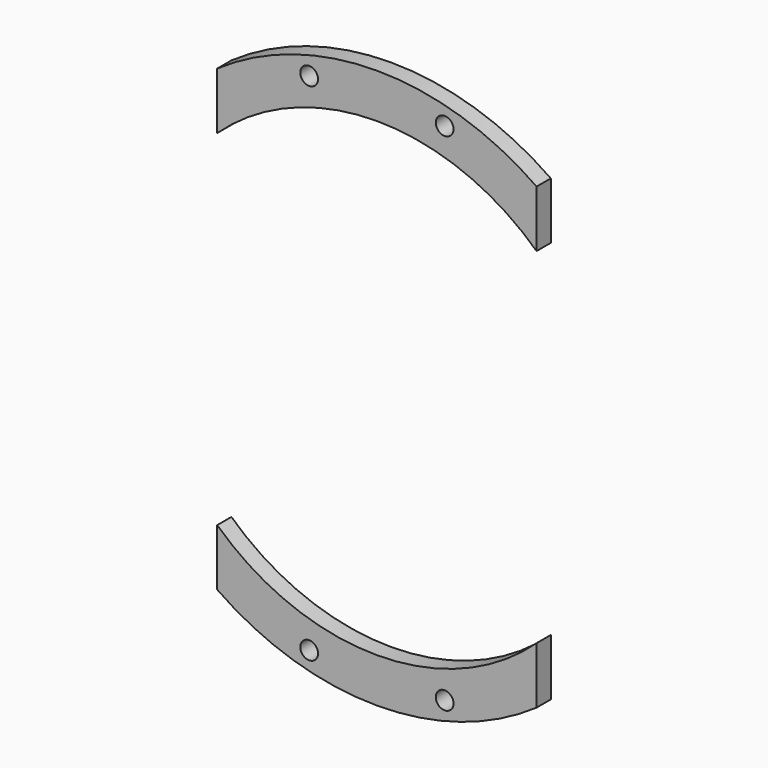
from build123d import *

# Parameters (mm, degrees)
F0_R     = 10
F1_DEPTH = 20


with BuildPart() as f1:
    # F0 (on Front) → F1 (new body)
    with BuildSketch(Plane.XZ):
        with BuildLine():
            ThreePointArc((-180, 194.4865033878), (0, 265), (180, 194.4865033878))
            Line((180, 194.4865033878), (180, 258.5053190942))
            ThreePointArc((180, 258.5053190942), (0, 315), (-180, 258.5053190942))
            Line((-180, 258.5053190942), (-180, 194.4865033878))
        make_face()
        with Locations((-76.3516183052, 284.9481187553)):
            Circle(F0_R, mode=Mode.SUBTRACT)
        with Locations((76.3516183052, 284.9481187553)):
            Circle(F0_R, mode=Mode.SUBTRACT)
    extrude(amount=F1_DEPTH)


with BuildPart() as f1b:
    # F0 (on Front) → F1, piece 2 (new body)
    with BuildSketch(Plane.XZ):
        with BuildLine():
            Line((180, -258.5053190942), (180, -194.4865033878))
            ThreePointArc((180, -194.4865033878), (0, -265), (-180, -194.4865033878))
            Line((-180, -194.4865033878), (-180, -258.5053190942))
            ThreePointArc((-180, -258.5053190942), (0, -315), (180, -258.5053190942))
        make_face()
        with Locations((-76.3516183052, -284.9481187553)):
            Circle(F0_R, mode=Mode.SUBTRACT)
        with Locations((76.3516183052, -284.9481187553)):
            Circle(F0_R, mode=Mode.SUBTRACT)
    extrude(amount=F1_DEPTH)


solid = Compound([f1.part, f1b.part])
